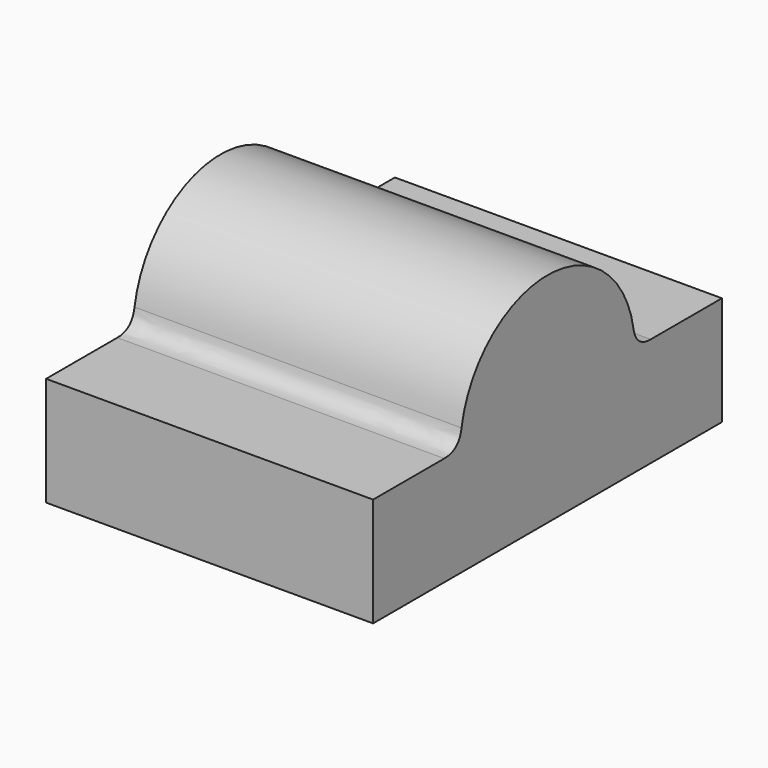
from build123d import *

# Parameters (mm, degrees)
F1_DEPTH    = 76.2
F2_T1_DEPTH = 76.2
F5_R        = 10.16


# Not quite as in the source:
# - a fillet or chamfer that OpenCascade refuses, or shapes differently, is made with other operations: its cross-section is extruded or revolved along the edge and cut away or added


with BuildPart() as f1:
    # F0 (on Right) → F1 (new body)
    with BuildSketch(Plane.YZ):
        with BuildLine():
            Line((-50.8, 0), (0, 0))
            Line((0, 0), (50.8, 0))
            Line((50.8, 0), (50.8, 25.4))
            Line((50.8, 25.4), (25.4, 25.4))
            ThreePointArc((25.4, 25.4), (0, 50.8), (-25.4, 25.4))
            Line((-25.4, 25.4), (-50.8, 25.4))
            Line((-50.8, 25.4), (-50.8, 0))
        make_face()
    extrude(amount=F1_DEPTH)

    # F2: fillet of radius 5.08 on 2 edges, made by hand

    # F2_s2 → F2_t1 (join)
    with BuildSketch(Plane.YZ):
        with BuildLine():
            add(Edge.make_bspline(
                [(-30.0536852981, 25.4), (-25.7603016841, 25.4), (-25.0447377485, 29.6333333333)],
                knots=[0, 0, 0, 1, 1, 1], degree=2, weights=[1, 1, 1]))
            ThreePointArc((-25.0447377485, 29.6333333333), (-25.3110286122, 27.5241070111), (-25.4, 25.4))
            Line((-25.4, 25.4), (-30.0536852981, 25.4))
        make_face()
        with BuildLine():
            add(Edge.make_bspline(
                [(30.0536852981, 25.4), (25.7603016841, 25.4), (25.0447377485, 29.6333333333)],
                knots=[0, 0, 0, 1, 1, 1], degree=2, weights=[1, 1, 1]))
            ThreePointArc((25.0447377485, 29.6333333333), (25.3110286122, 27.5241070111), (25.4, 25.4))
            Line((25.4, 25.4), (30.0536852981, 25.4))
        make_face()
    extrude(amount=F2_T1_DEPTH)

    # F3 (on face) → F4 (revolve, cut)
    with BuildSketch(Plane(origin=(0, 0, 0), x_dir=(0, -1, 0), z_dir=(-1, 0, 0))):
        with BuildLine():
            Line((0, 45.441377908), (0, 3.5084052943))
            Line((0, 3.5084052943), (45.9408350289, 3.5084052943))
            Line((45.9408350289, 3.5084052943), (45.9408350289, 17.5937116146))
            Line((45.9408350289, 17.5937116146), (18.4585668484, 17.5937116146))
            ThreePointArc((18.4585668484, 17.5937116146), (16.7048736009, 36.4726702484), (0, 45.441377908))
        make_face()
    revolve(axis=Axis((0, 0, 24.4748916011), (0, 0, -1)), mode=Mode.SUBTRACT)

    # F5
    f5_edges = [f1.edges().sort_by_distance(p)[0] for p in [
        (18.458567, 0, 17.593712),
    ]]
    fillet(f5_edges, radius=F5_R)


solid = f1.part
